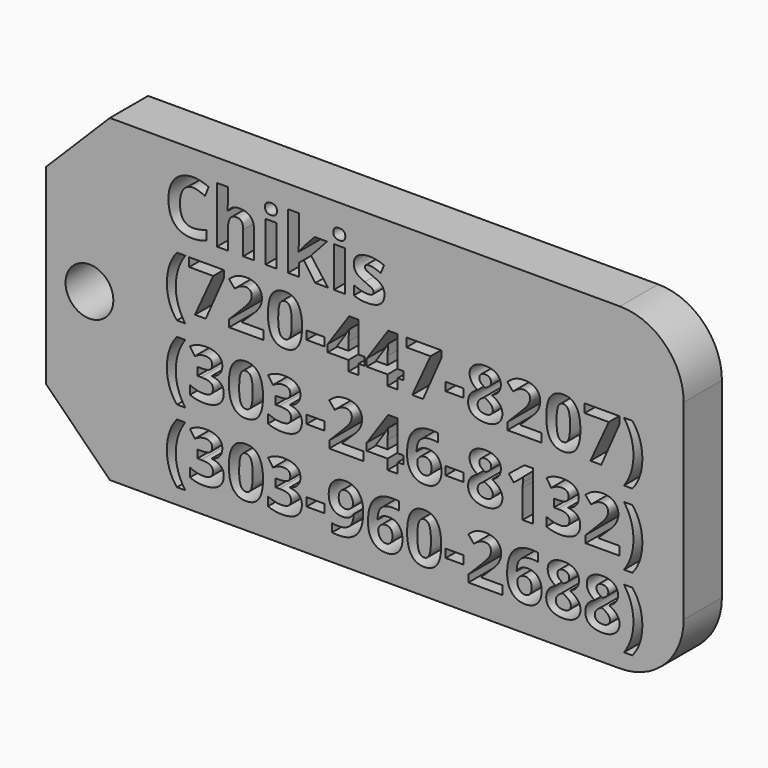
from build123d import *

# Parameters (mm, degrees)
F0_W           = 50.8
F0_H           = 25.4
F1_DEPTH       = 3.81
F2_SIZE        = 5.08
F3_R           = 5.08
F5_R           = 1.905
F6_DEPTH       = 25.4
F7_TEXT_SIZE   = 5.8817466201
F7_TEXT_SIZE_2 = 5.4513749162
F8_DEPTH       = 3.811


# Not quite as in the source:
# - Text() gives the source's letters only with a copy of the font that has no kerning and outlines rounded to 1/6400 em; it was checked with that copy


with BuildPart() as f1:
    # F0 (on Front) → F1 (new body)
    with BuildSketch(Plane.XZ):
        with Locations((-2.7113604963, -13.3525603144)):
            Rectangle(F0_W, F0_H)
    extrude(amount=F1_DEPTH)

    # F2
    f2_edges = [f1.edges().sort_by_distance(p)[0] for p in [
        (-28.11136, -1.905, -0.65256),
        (-28.11136, -1.905, -26.05256),
    ]]
    chamfer(f2_edges, length=F2_SIZE)

    # F3
    f3_edges = [f1.edges().sort_by_distance(p)[0] for p in [
        (22.68864, -1.905, -0.65256),
        (22.68864, -1.905, -26.05256),
    ]]
    fillet(f3_edges, radius=F3_R)

    # F5 (on face) → F6 (cut)
    with BuildSketch(Plane.XZ.offset(3.81)):
        with Locations((-24.6564522386, -13.3525603144)):
            Circle(F5_R)
    extrude(amount=-F6_DEPTH, mode=Mode.SUBTRACT)

    # F7 (on face) → F8 (cut, through all)
    with BuildSketch(Plane.XZ.offset(3.81)):
        with Locations((-18.7032236022, -6.9040756125)):
            Text('Chikis', F7_TEXT_SIZE, font='Open Sans', font_style=FontStyle.BOLD, text_align=(TextAlign.LEFT, TextAlign.BOTTOM))
        with Locations((-18.7032236022, -12.2498747864)):
            Text('(720-447-8207)', F7_TEXT_SIZE_2, font='Open Sans', font_style=FontStyle.BOLD, text_align=(TextAlign.LEFT, TextAlign.BOTTOM))
        with Locations((-18.7032236022, -18.155970406)):
            Text('(303-246-8132)', F7_TEXT_SIZE_2, font='Open Sans', font_style=FontStyle.BOLD, text_align=(TextAlign.LEFT, TextAlign.BOTTOM))
        with Locations((-18.7032236022, -23.9488421107)):
            Text('(303-960-2688)', F7_TEXT_SIZE_2, font='Open Sans', font_style=FontStyle.BOLD, text_align=(TextAlign.LEFT, TextAlign.BOTTOM))
    extrude(amount=-F8_DEPTH, mode=Mode.SUBTRACT)


solid = f1.part
